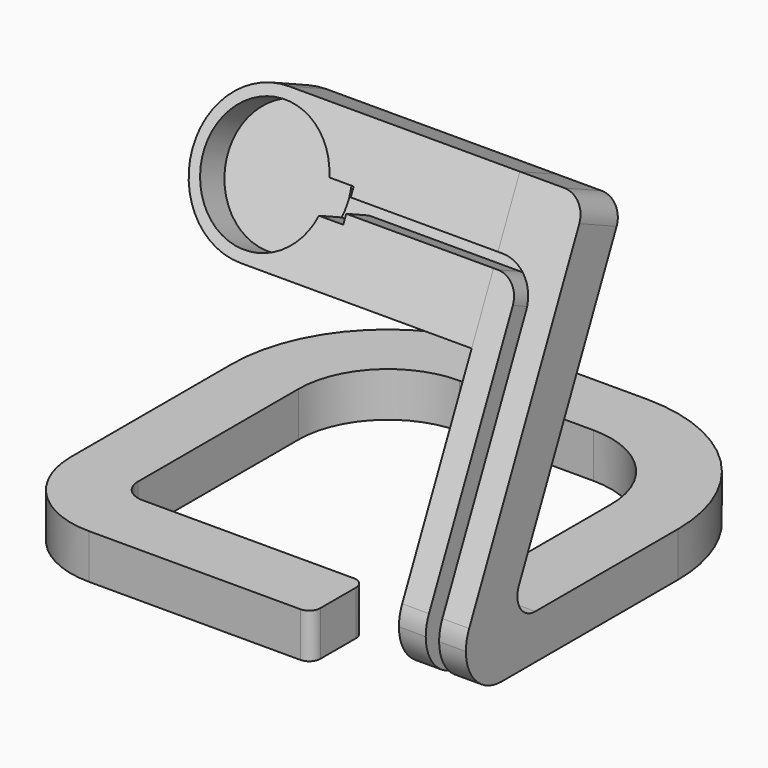
from build123d import *

# Parameters (mm, degrees)
F1_DEPTH  = 10
F3_DEPTH  = 25.0000003725
F4_DEPTH  = 15
F5_R      = 13.75
F6_DEPTH  = 11.5
F7_DEPTH  = 7.5
F8_W      = 3
F8_H      = 12.169879545
F9_DEPTH  = 7
F10_W     = 3
F10_H     = 7.9815720619
F11_DEPTH = 4
F12_R     = 5
F13_R     = 5


# Not quite as in the source:
# - a feature names something its author has since deleted; it is built from what else it names


with BuildPart() as f1:
    # F0 (on Top) → F1 (new body)
    with BuildSketch(Plane.XY):
        with BuildLine():
            ThreePointArc((50, 15), (39.7487373415, 39.7487373415), (15, 50))
            Line((15, 50), (-15, 50))
            ThreePointArc((-15, 50), (-39.7487373415, 39.7487373415), (-50, 15))
            Line((-50, 15), (-50, -30))
            ThreePointArc((-50, -30), (-44.1421356237, -44.1421356237), (-30, -50))
            Line((-30, -50), (17.3621465266, -50))
            ThreePointArc((17.3621465266, -50), (19.1299134795, -49.267766953), (19.8621465266, -47.5))
            Line((19.8621465266, -47.5), (19.8621465266, -37.5))
            ThreePointArc((19.8621465266, -37.5), (19.1299134795, -35.732233047), (17.3621465266, -35))
            Line((17.3621465266, -35), (-30, -35))
            ThreePointArc((-30, -35), (-33.5355339059, -33.5355339059), (-35, -30))
            Line((-35, -30), (-35, 15))
            ThreePointArc((-35, 15), (-29.1421356237, 29.1421356237), (-15, 35))
            Line((-15, 35), (15, 35))
            ThreePointArc((15, 35), (29.1421356237, 29.1421356237), (35, 15))
            Line((35, 15), (35, -35))
            Line((35, -35), (35, -50))
            Line((35, -50), (50, -50))
            Line((50, -50), (50, 15))
        make_face()
    extrude(amount=F1_DEPTH)

    # F2 (on face) → F3 (cut)
    with BuildSketch(Plane.YZ.offset(50)):
        with BuildLine():
            ThreePointArc((-34.4148690401, 0), (-41.4859368519, 2.9289321881), (-44.4148690401, 10))
            Line((-44.4148690401, 10), (-50, 10))
            Line((-50, 10), (-50, 0))
            Line((-50, 0), (-34.4148690401, 0))
        make_face()
    extrude(amount=-F3_DEPTH, mode=Mode.SUBTRACT)

    # F2 (on face) → F4 (join)
    with BuildSketch(Plane.YZ.offset(50)):
        with BuildLine():
            Line((-10.5677563486, 86.0143546169), (-43.5051570601, 14.1673329256))
            ThreePointArc((-43.5051570601, 14.1673329256), (-44.1847943264, 12.1327353094), (-44.4148690401, 10))
            Line((-44.4148690401, 10), (-24.9867949218, 10))
            ThreePointArc((-24.9867949218, 10), (-29.1950209325, 12.299845589), (-29.5319389318, 17.0836664628))
            Line((-29.5319389318, 17.0836664628), (-0.1259929755, 81.2274541128))
            Line((-0.1259929755, 81.2274541128), (-10.5677563486, 86.0143546169))
        make_face()
    extrude(amount=-F4_DEPTH)

    # F5 (on face) → F6 (join)
    with BuildSketch(Plane(origin=(0, -41.3166681437, 18.9411282845), x_dir=(1, 0, 0), z_dir=(0, -0.909028802, 0.4167332926))):
        with BuildLine():
            ThreePointArc((-0.5725613731, 57.6122225326), (-5.3096309812, 69.0485202264), (-16.7459286749, 73.7855898345))
            ThreePointArc((-16.7459286749, 73.7855898345), (-32.9192959768, 57.6122225326), (-16.7459286749, 41.4388552308))
            ThreePointArc((-16.7459286749, 41.4388552308), (-5.3096309812, 46.1759248389), (-0.5725613731, 57.6122225326))
        make_face()
        with Locations((-16.7459286749, 57.6122225326)):
            Circle(F5_R, mode=Mode.SUBTRACT)
        with Locations((-16.7459286749, 57.6122225326)):
            Circle(F5_R)
        with BuildLine():
            Line((35, 41.4388552308), (35, 73.7855898345))
            Line((35, 73.7855898345), (-16.7459286749, 73.7855898345))
            ThreePointArc((-16.7459286749, 73.7855898345), (-5.3096309812, 69.0485202264), (-0.5725613731, 57.6122225326))
            ThreePointArc((-0.5725613731, 57.6122225326), (-5.3096309812, 46.1759248389), (-16.7459286749, 41.4388552308))
            Line((-16.7459286749, 41.4388552308), (35, 41.4388552308))
        make_face()
    extrude(amount=-F6_DEPTH)

    # F5 (on face) → F7 (cut)
    with BuildSketch(Plane(origin=(0, -41.3166681437, 18.9411282845), x_dir=(1, 0, 0), z_dir=(0, -0.909028802, 0.4167332926))):
        with Locations((-16.7459286749, 57.6122225326)):
            Circle(F5_R)
    extrude(amount=-F7_DEPTH, mode=Mode.SUBTRACT)

    # F8 (on face) → F9 (cut)
    with BuildSketch(Plane(origin=(0, -41.3166681437, 18.9411282845), x_dir=(1, 0, 0), z_dir=(0, -0.909028802, 0.4167332926))):
        with BuildLine():
            Line((2.0040713251, 56.1122225326), (2.0040713251, 59.1122225326))
            Line((2.0040713251, 59.1122225326), (2.0040713251, 61.1122225326))
            Line((2.0040713251, 61.1122225326), (-3.448842528, 61.1122225326))
            ThreePointArc((-3.448842528, 61.1122225326), (-3.109627224, 59.376813913), (-2.9959286749, 57.6122225326))
            ThreePointArc((-2.9959286749, 57.6122225326), (-3.109627224, 55.8476311523), (-3.448842528, 54.1122225326))
            Line((-3.448842528, 54.1122225326), (2.0040713251, 54.1122225326))
            Line((2.0040713251, 54.1122225326), (2.0040713251, 56.1122225326))
        make_face()
        with BuildLine():
            Line((36, 59.1122225326), (2.0040713251, 59.1122225326))
            Line((2.0040713251, 59.1122225326), (2.0040713251, 56.1122225326))
            Line((2.0040713251, 56.1122225326), (36, 56.1122225326))
            ThreePointArc((36, 56.1122225326), (39.5355339059, 54.6477564386), (41, 51.1122225326))
            Line((41, 51.1122225326), (41, -5.251533668))
            Line((41, -5.251533668), (44, -5.251533668))
            Line((44, -5.251533668), (44, 51.1122225326))
            ThreePointArc((44, 51.1122225326), (41.6568542495, 56.7690767821), (36, 59.1122225326))
        make_face()
        with Locations((42.5, -11.3364734405)):
            Rectangle(F8_W, F8_H)
    extrude(amount=-F9_DEPTH, mode=Mode.SUBTRACT)

    # F10 (on face) → F11 (cut)
    with BuildSketch(Plane(origin=(0, 0, 0), x_dir=(1, 0, 0), z_dir=(0, 0, -1))):
        with Locations((42.5, 38.4056550711)):
            Rectangle(F10_W, F10_H)
        with BuildLine():
            Line((44, 34.4148690401), (41, 34.4148690401))
            Line((41, 34.4148690401), (41, -38.4307490277))
            ThreePointArc((41, -38.4307490277), (42.5667640895, -36.5655632349), (44, -34.5959179423))
            Line((44, -34.5959179423), (44, 34.4148690401))
        make_face()
    extrude(amount=-F11_DEPTH, mode=Mode.SUBTRACT)

    # F12
    f12_edges = [f1.edges().sort_by_distance(p)[0] for p in [
        (42.5, -40.465722, 4),
    ]]
    fillet(f12_edges, radius=F12_R)

    # F13
    f13_edges = [f1.edges().sort_by_distance(p)[0] for p in [
        (50, -5.346875, 83.620904),
    ]]
    fillet(f13_edges, radius=F13_R)


solid = f1.part
